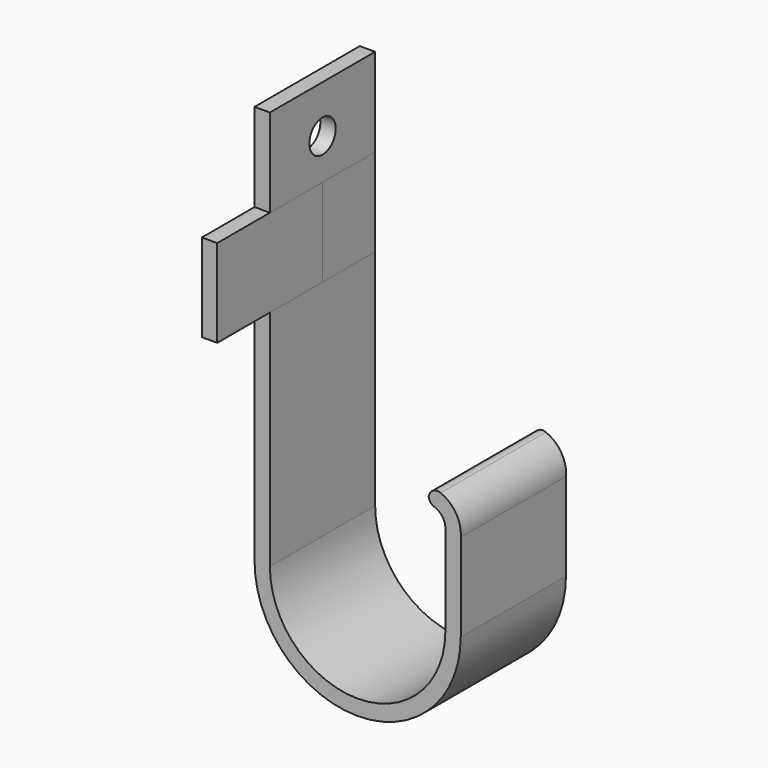
from build123d import *

# Parameters (mm, degrees)
F0_W        = 3.5
F0_H        = 20.1132470577
F1_DEPTH    = 15
F0_H_2      = 21.1232600108
F0_H_3      = 29.8616039545
F3_D        = 7.5
F4_T1_DEPTH = 38.2360477135
F4_T3_DEPTH = 43.9936648007
F5_DEPTH    = 30
F6_DEPTH    = 15


# Not quite as in the source:
# - a fillet or chamfer that OpenCascade refuses, or shapes differently, is made with other operations: its cross-section is extruded or revolved along the edge and cut away or added


with BuildPart() as f1:
    # F0 (on Front) → F1 (new body, symmetric)
    with BuildSketch(Plane.XZ):
        with Locations((-22.3977046013, 89.9042797192)):
            Rectangle(F0_W, F0_H)
    extrude(amount=F1_DEPTH, both=True)

    # F3 (through all)
    with Locations(Plane.YZ):
        with Locations((0, 89.1436196168)):
            Hole(F3_D / 2)


with BuildPart() as f1b:
    # F0 (on Front) → F1, piece 2 (new body, symmetric)
    with BuildSketch(Plane.XZ):
        with Locations((-22.3977046013, 19.3992732427)):
            Rectangle(F0_W, F0_H_2)
        with BuildLine():
            Line((-20.6477046013, 8.8376432372), (-24.1477046013, 8.8376432372))
            ThreePointArc((-24.1477046013, 8.8376432372), (-0.6477046013, -14.6623567628), (22.8522953987, 8.8376432372))
            Line((22.8522953987, 8.8376432372), (19.3522953987, 8.8376432372))
            ThreePointArc((19.3522953987, 8.8376432372), (-0.6477046013, -11.1623567628), (-20.6477046013, 8.8376432372))
        make_face()
        Polygon((19.3522953987, 8.8376432372), (22.8522953987, 8.8376432372), (22.8696210889, 8.8376432372), (22.8696210889, 28.8880299777), (19.3522953987, 28.8880299777), align=None)
        with BuildLine():
            ThreePointArc((15.540712513, 33.2429967821), (18.4344082452, 31.930153514), (19.3522953987, 28.8880299777))
            Line((19.3522953987, 28.8880299777), (22.8696210889, 28.8880299777))
            ThreePointArc((22.8696210889, 28.8880299777), (20.9352317559, 34.4482994471), (15.540712513, 36.8057601154))
            Line((15.540712513, 36.8057601154), (15.540712513, 33.2429967821))
        make_face()
        with Locations((-22.3977046013, 44.8917052254)):
            Rectangle(F0_W, F0_H_3)
    extrude(amount=F1_DEPTH, both=True)

    # F4: fillet of radius 2 on 2 edges, made by hand

    # F4_s2 → F4_t1 (cut)
    with BuildSketch(Plane.XZ.offset(-19.1180238568)):
        with BuildLine():
            ThreePointArc((16.8564234422, 33.0109116519), (15.9023324989, 33.7431618927), (15.540712513, 34.8902063248))
            Line((15.540712513, 34.8902063248), (15.540712513, 33.2429967821))
            ThreePointArc((15.540712513, 33.2429967821), (16.2087242563, 33.1845310505), (16.8564234422, 33.0109116519))
        make_face()
    extrude(amount=F4_T1_DEPTH, mode=Mode.SUBTRACT)

    # F4_s4 → F4_t3 (cut)
    with BuildSketch(Plane.XZ.offset(-21.9968324004)):
        with BuildLine():
            ThreePointArc((15.540712513, 34.4179292964), (16.4215839799, 36.0755032243), (18.2882638394, 36.2729675749))
            ThreePointArc((18.2882638394, 36.2729675749), (16.9400789931, 36.6713328153), (15.540712513, 36.8057601154))
            Line((15.540712513, 36.8057601154), (15.540712513, 34.4179292964))
        make_face()
    extrude(amount=F4_T3_DEPTH, mode=Mode.SUBTRACT)


with BuildPart() as f5:
    # F0 (on Front) → F5 (new body)
    with BuildSketch(Plane.XZ):
        Polygon((-20.6477046013, 79.8476561904), (-24.1477046013, 79.8476561904), (-24.1477046013, 59.8225072026), (-20.6477046013, 59.8225072026), (-20.6477046013, 65.9805735738), align=None)
    extrude(amount=F5_DEPTH)


with BuildPart() as f6:
    # F0 (on Front) → F6 (new body)
    with BuildSketch(Plane.XZ):
        Polygon((-20.6477046013, 79.8476561904), (-24.1477046013, 79.8476561904), (-24.1477046013, 59.8225072026), (-20.6477046013, 59.8225072026), (-20.6477046013, 65.9805735738), align=None)
    extrude(amount=-F6_DEPTH)


solid = Compound([f1.part, f1b.part, f5.part, f6.part])
